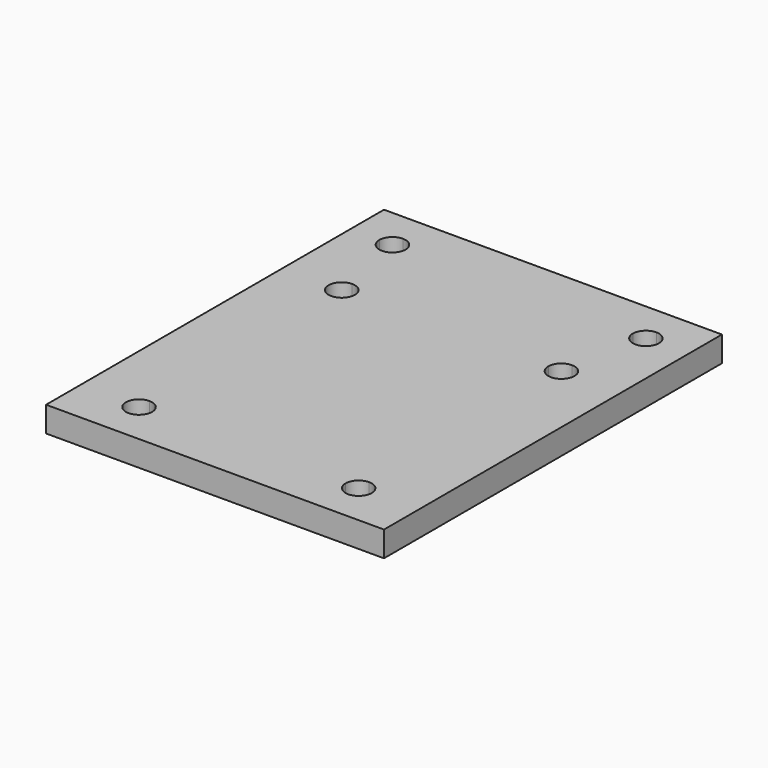
from build123d import *

# Parameters (mm, degrees)
F0_W     = 16
F0_H     = 5
F1_DEPTH = 3
F2_DEPTH = 5
F3_SIZE  = 4.99999


# Not quite as in the source:
# - a fillet or chamfer is up to 0.001 mm smaller than in the source, because OpenCascade refuses the exact size


with BuildPart() as f1:
    # F0 (on Top) → F1 (new body)
    with BuildSketch(Plane.XY):
        with BuildLine():
            ThreePointArc((-13, -13.45), (-11.9039844892, -13.9039844892), (-11.45, -15))
            Line((-11.45, -15), (11.45, -15))
            ThreePointArc((11.45, -15), (11.9039844892, -13.9039844892), (13, -13.45))
            Line((13, -13.45), (13, 13.45))
            ThreePointArc((13, 13.45), (11.9039844892, 13.9039844892), (11.45, 15))
            Line((11.45, 15), (8, 15))
            Line((8, 15), (-8, 15))
            Line((-8, 15), (-11.45, 15))
            ThreePointArc((-11.45, 15), (-11.9039844892, 13.9039844892), (-13, 13.45))
            Line((-13, 13.45), (-13, -13.45))
        make_face()
        with BuildLine():
            Line((11.45, -15), (-11.45, -15))
            ThreePointArc((-11.45, -15), (-14.0960155108, -16.0960155108), (-13, -13.45))
            Line((-13, -13.45), (-13, 13.45))
            ThreePointArc((-13, 13.45), (-14.55, 15), (-13, 16.55))
            Line((-13, 16.55), (-13, 20))
            Line((-13, 20), (-20, 20))
            Line((-20, 20), (-20, -20))
            Line((-20, -20), (20, -20))
            Line((20, -20), (20, 20))
            Line((20, 20), (13, 20))
            Line((13, 20), (13, 16.55))
            ThreePointArc((13, 16.55), (14.0960155108, 16.0960155108), (14.55, 15))
            ThreePointArc((14.55, 15), (14.0960155108, 13.9039844892), (13, 13.45))
            Line((13, 13.45), (13, -13.45))
            ThreePointArc((13, -13.45), (14.0960155108, -13.9039844892), (14.55, -15))
            ThreePointArc((14.55, -15), (13, -16.55), (11.45, -15))
        make_face()
        with BuildLine():
            Line((-13, 20), (-13, 16.55))
            ThreePointArc((-13, 16.55), (-11.9039844892, 16.0960155108), (-11.45, 15))
            Line((-11.45, 15), (-8, 15))
            Line((-8, 15), (-8, 20))
            Line((-8, 20), (-13, 20))
        make_face()
        with BuildLine():
            Line((8, 15), (11.45, 15))
            ThreePointArc((11.45, 15), (11.9039844892, 16.0960155108), (13, 16.55))
            Line((13, 16.55), (13, 20))
            Line((13, 20), (8, 20))
            Line((8, 20), (8, 15))
        make_face()
        with BuildLine():
            Line((-20, 20), (-13, 20))
            Line((-13, 20), (-8, 20))
            Line((-8, 20), (8, 20))
            Line((8, 20), (13, 20))
            Line((13, 20), (20, 20))
            Line((20, 20), (20, 30))
            Line((20, 30), (15, 30))
            Line((15, 30), (15, 26.55))
            ThreePointArc((15, 26.55), (16.0960155108, 26.0960155108), (16.55, 25))
            ThreePointArc((16.55, 25), (15, 23.45), (13.45, 25))
            Line((13.45, 25), (-13.45, 25))
            ThreePointArc((-13.45, 25), (-15, 23.45), (-16.55, 25))
            Line((-16.55, 25), (-20, 25))
            Line((-20, 25), (-20, 20))
        make_face()
        with Locations((0, 17.5)):
            Rectangle(F0_W, F0_H)
        with BuildLine():
            Line((-20, 30), (-20, 25))
            Line((-20, 25), (-16.55, 25))
            ThreePointArc((-16.55, 25), (-16.0960155108, 26.0960155108), (-15, 26.55))
            Line((-15, 26.55), (-15, 30))
            Line((-15, 30), (-20, 30))
        make_face()
        with BuildLine():
            Line((15, 30), (-15, 30))
            Line((-15, 30), (-15, 26.55))
            ThreePointArc((-15, 26.55), (-13.9039844892, 26.0960155108), (-13.45, 25))
            Line((-13.45, 25), (13.45, 25))
            ThreePointArc((13.45, 25), (13.9039844892, 26.0960155108), (15, 26.55))
            Line((15, 26.55), (15, 30))
        make_face()
    extrude(amount=F1_DEPTH)

    # F0 (on Top) → F2 (join)
    with BuildSketch(Plane.XY):
        with Locations((0, 17.5)):
            Rectangle(F0_W, F0_H)
    extrude(amount=-F2_DEPTH)

    # F3 (size 5 in the source; OpenCascade refuses exactly that, so slightly less here)
    f3_edges = [f1.edges().sort_by_distance(p)[0] for p in [
        (0, 15, -5),
    ]]
    chamfer(f3_edges, length=F3_SIZE)


solid = f1.part
